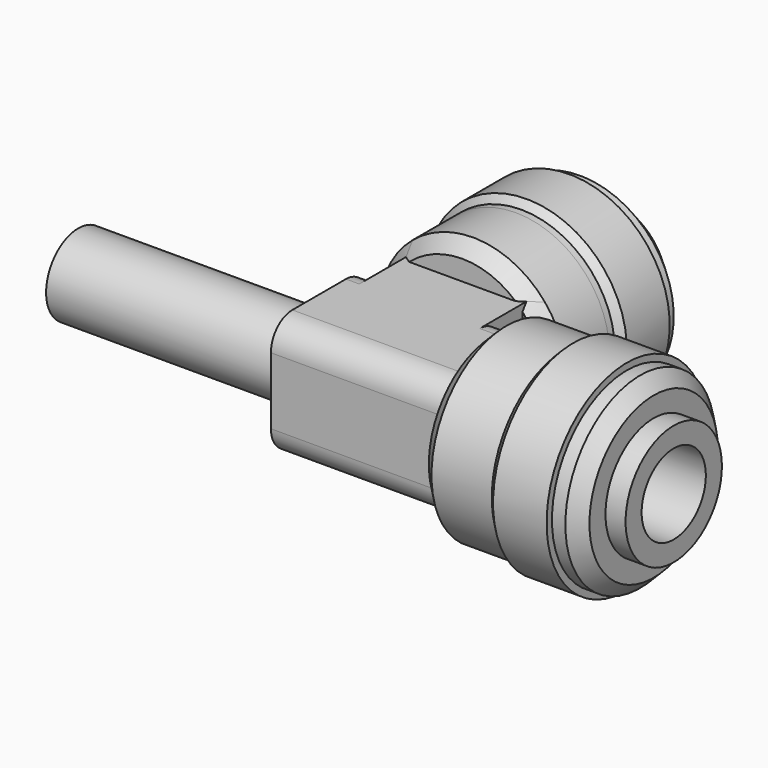
from build123d import *

# Parameters (mm, degrees)
F1_DEPTH     = 9
F2_R         = 2
F3_R         = 3
F3_R_2       = 2
F4_DEPTH     = 18
F5_R         = 7
F6_DEPTH     = 5
F8_R         = 7.5
F9_DEPTH     = 5
F10_S5_R     = 7
F10_T6_DEPTH = 12
F11_R        = 7
F12_DEPTH    = 2
F13_SIZE     = 1
F14_R        = 4.5
F15_DEPTH    = 1.5
F16_R        = 3
F17_DEPTH    = 15
F18_R        = 7
F19_DEPTH    = 5
F20_R        = 7.5
F21_DEPTH    = 5
F22_R        = 7
F23_DEPTH    = 2
F24_R        = 4.5
F25_DEPTH    = 1.5
F26_R        = 3
F27_DEPTH    = 25
F28_S7_R     = 7
F28_T8_DEPTH = 12


# Not quite as in the source:
# - a fillet or chamfer that OpenCascade refuses, or shapes differently, is made with other operations: its cross-section is extruded or revolved along the edge and cut away or added
# - a feature names something its author has since deleted; it is built from what else it names


with BuildPart() as f1:
    # F0 (on Top) → F1 (new body)
    with BuildSketch(Plane.XY):
        Polygon((-10, -4.5), (3, -4.5), (3, 4.5), (0, 4.5), (0, 6.5), (-9, 6.5), (-9, 4.5), (-10, 4.5), align=None)
    extrude(amount=F1_DEPTH)

    # F2
    f2_edges = [f1.edges().sort_by_distance(p)[0] for p in [
        (-3.5, -4.5, 9),
        (-3.5, -4.5, 0),
        (1.5, 4.5, 0),
        (1.5, 4.5, 9),
        (-9.5, 4.5, 9),
        (-9.5, 4.5, 0),
    ]]
    fillet(f2_edges, radius=F2_R)

    # F3 (on face) → F4 (join)
    with BuildSketch(Plane(origin=(-10, 0, 0), x_dir=(0, -1, 0), z_dir=(-1, 0, 0))):
        with Locations((0, 4.5)):
            Circle(F3_R)
        with Locations((0, 4.5)):
            Circle(F3_R_2, mode=Mode.SUBTRACT)
    extrude(amount=F4_DEPTH)

    # F5 (on face) → F6 (join)
    with BuildSketch(Plane(origin=(0, 6.5, 0), x_dir=(-1, 0, 0), z_dir=(0, 1, 0))):
        with Locations((4.5, 4.5)):
            Circle(F5_R)
    extrude(amount=F6_DEPTH)

    # F7: chamfer of 1 on 1 edges, made by hand


with BuildPart() as f7_tool2:
    # F7_s3 → F7_t4 (revolve)
    with BuildSketch(Plane.XY.offset(4.5)):
        Polygon((-11.5, 7.5), (-10.5, 6.5), (-11.5, 6.5), align=None)
    revolve(axis=Axis((-4.5, 6.5, 4.5), (0, 1, 0)))

    split(bisect_by=Plane.YZ.offset(-9), keep=Keep.BOTTOM)


with BuildPart() as f1_1:
    add(f1.part)

    # F7_t1: cut F7_tool2
    add(f7_tool2.part, mode=Mode.SUBTRACT)


with BuildPart() as f7_tool7:
    # F7_s8 → F7_t9 (revolve)
    with BuildSketch(Plane.XY.offset(4.5)):
        Polygon((-11.5, 7.5), (-10.5, 6.5), (-11.5, 6.5), align=None)
    revolve(axis=Axis((-4.5, 6.5, 4.5), (0, 1, 0)))

    split(bisect_by=Plane.XY.offset(9), keep=Keep.TOP)


with BuildPart() as f1_2:
    add(f1_1.part)

    # F7_t6: cut F7_tool7
    add(f7_tool7.part, mode=Mode.SUBTRACT)


with BuildPart() as f7_tool12:
    # F7_s13 → F7_t14 (revolve)
    with BuildSketch(Plane.XY.offset(4.5)):
        Polygon((-11.5, 7.5), (-10.5, 6.5), (-11.5, 6.5), align=None)
    revolve(axis=Axis((-4.5, 6.5, 4.5), (0, 1, 0)))

    split(bisect_by=Plane.XY, keep=Keep.BOTTOM)


with BuildPart() as f1_3:
    add(f1_2.part)

    # F7_t11: cut F7_tool12
    add(f7_tool12.part, mode=Mode.SUBTRACT)


with BuildPart() as f7_tool17:
    # F7_s18 → F7_t19 (revolve)
    with BuildSketch(Plane.XY.offset(4.5)):
        Polygon((-11.5, 7.5), (-10.5, 6.5), (-11.5, 6.5), align=None)
    revolve(axis=Axis((-4.5, 6.5, 4.5), (0, 1, 0)))

    split(bisect_by=Plane.YZ, keep=Keep.TOP)


with BuildPart() as f1_4:
    add(f1_3.part)

    # F7_t16: cut F7_tool17
    add(f7_tool17.part, mode=Mode.SUBTRACT)

    # F8 (on face) → F9 (join)
    with BuildSketch(Plane(origin=(0, 11.5, 0), x_dir=(-1, 0, 0), z_dir=(0, 1, 0))):
        with Locations((4.5, 4.5)):
            Circle(F8_R)
    extrude(amount=F9_DEPTH)

    # F10: chamfer of 1 on 1 edges, made by hand


with BuildPart() as f10_tool2:
    # F10_s3 → F10_t4 (revolve)
    with BuildSketch(Plane.XY.offset(4.5)):
        Polygon((-12, 12.5), (-11, 11.5), (-12, 11.5), align=None)
    revolve(axis=Axis((-4.5, 11.5, 4.5), (0, 1, 0)))

    # F10_s5 → F10_t6 (cut, symmetric)
    with BuildSketch(Plane.XZ.offset(-12)):
        with Locations((-4.5, 4.5)):
            Circle(F10_S5_R)
    extrude(amount=F10_T6_DEPTH, both=True, mode=Mode.SUBTRACT)


with BuildPart() as f1_5:
    add(f1_4.part)

    # F10_t1: cut F10_tool2
    add(f10_tool2.part, mode=Mode.SUBTRACT)

    # F11 (on face) → F12 (join)
    with BuildSketch(Plane(origin=(0, 16.5, 0), x_dir=(-1, 0, 0), z_dir=(0, 1, 0))):
        with Locations((4.5, 4.5)):
            Circle(F11_R)
    extrude(amount=F12_DEPTH)

    # F13
    f13_edges = [f1_5.edges().sort_by_distance(p)[0] for p in [
        (2.5, 18.5, 4.5),
    ]]
    chamfer(f13_edges, length=F13_SIZE)

    # F14 (on face) → F15 (join)
    with BuildSketch(Plane(origin=(0, 18.5, 0), x_dir=(-1, 0, 0), z_dir=(0, 1, 0))):
        with Locations((4.5, 4.5)):
            Circle(F14_R)
    extrude(amount=F15_DEPTH)

    # F16 (on face) → F17 (cut)
    with BuildSketch(Plane(origin=(0, 20, 0), x_dir=(-1, 0, 0), z_dir=(0, 1, 0))):
        with Locations((4.5, 4.5)):
            Circle(F16_R)
    extrude(amount=-F17_DEPTH, mode=Mode.SUBTRACT)

    # F18 (on face) → F19 (join)
    with BuildSketch(Plane.YZ.offset(3)):
        with Locations((0, 4.5)):
            Circle(F18_R)
    extrude(amount=F19_DEPTH)

    # F20 (on face) → F21 (join)
    with BuildSketch(Plane.YZ.offset(8)):
        with Locations((0, 4.5)):
            Circle(F20_R)
    extrude(amount=F21_DEPTH)

    # F22 (on face) → F23 (join)
    with BuildSketch(Plane.YZ.offset(13)):
        with Locations((0, 4.5)):
            Circle(F22_R)
    extrude(amount=F23_DEPTH)

    # F24 (on face) → F25 (join)
    with BuildSketch(Plane.YZ.offset(15)):
        with Locations((0, 4.5)):
            Circle(F24_R)
    extrude(amount=F25_DEPTH)

    # F26 (on face) → F27 (cut)
    with BuildSketch(Plane.YZ.offset(16.5)):
        with Locations((0, 4.5)):
            Circle(F26_R)
    extrude(amount=-F27_DEPTH, mode=Mode.SUBTRACT)

    # F28: chamfer of 1 on 3 edges, made by hand

    # F28_s1 → F28_t2 (revolve, cut)
    with BuildSketch(Plane.XY.offset(4.5)):
        Polygon((4, 7), (3, 6), (3, 7), align=None)
    revolve(axis=Axis((3, 0, 4.5), (1, 0, 0)), mode=Mode.SUBTRACT)


with BuildPart() as f28_tool4:
    # F28_s5 → F28_t6 (revolve)
    with BuildSketch(Plane.XY.offset(4.5)):
        Polygon((9, 7.5), (8, 6.5), (8, 7.5), align=None)
    revolve(axis=Axis((8, 0, 4.5), (1, 0, 0)))

    # F28_s7 → F28_t8 (cut, symmetric)
    with BuildSketch(Plane.YZ.offset(8.5)):
        with Locations((0, 4.5)):
            Circle(F28_S7_R)
    extrude(amount=F28_T8_DEPTH, both=True, mode=Mode.SUBTRACT)


with BuildPart() as f1_6:
    add(f1_5.part)

    # F28_t3: cut F28_tool4
    add(f28_tool4.part, mode=Mode.SUBTRACT)

    # F28_s9 → F28_t10 (revolve, cut)
    with BuildSketch(Plane.XY.offset(4.5)):
        Polygon((14, 7), (15, 6), (15, 7), align=None)
    revolve(axis=Axis((15, 0, 4.5), (1, 0, 0)), mode=Mode.SUBTRACT)


solid = f1_6.part
